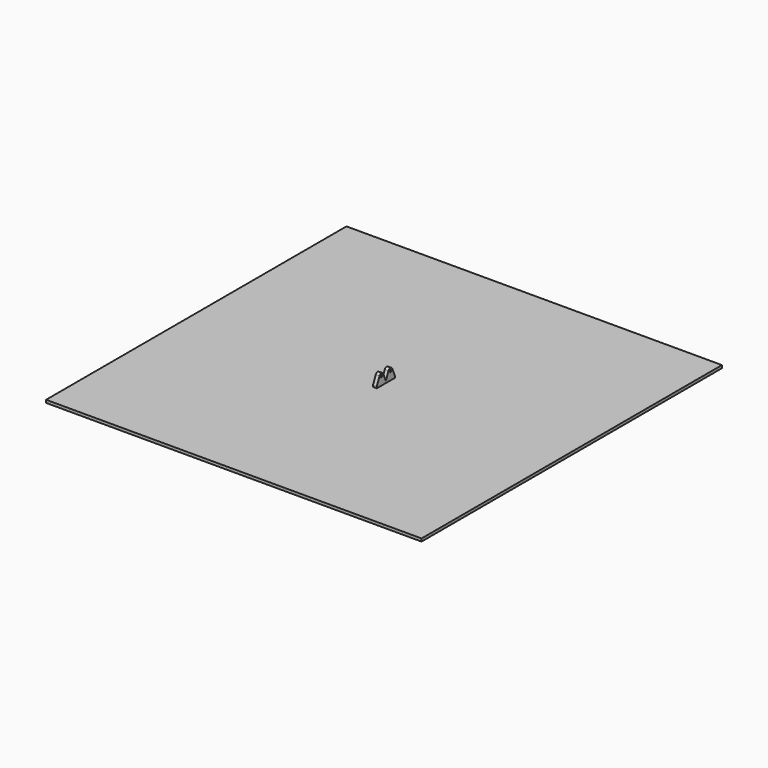
from build123d import *

# Parameters (mm, degrees)
F0_W     = 400
F0_H     = 400
F1_DEPTH = 3
F2_R     = 1.25
F2_W     = 12
F2_H     = 2
F3_DEPTH = 2
F4_DEPTH = 2


with BuildPart() as f1:
    # F0 (on Top) → F1 (new body)
    with BuildSketch(Plane.XY):
        Rectangle(F0_W, F0_H)
    extrude(amount=-F1_DEPTH)

    # F2 (on Right) → F3 (join)
    with BuildSketch(Plane.YZ):
        with BuildLine():
            ThreePointArc((-3.4732674635, 10.0854136027), (-6, 11.75), (-8.5267325365, 10.0854136027))
            ThreePointArc((-8.5267325365, 10.0854136027), (-6.5540692757, 6.3063951222), (-3.25, 9))
            ThreePointArc((-3.25, 9), (-3.3063951222, 9.5540692757), (-3.4732674635, 10.0854136027))
        make_face()
        with Locations((-6, 9)):
            Circle(F2_R, mode=Mode.SUBTRACT)
        with BuildLine():
            Line((-8.5267325365, 10.0854136027), (-12, 2))
            Line((-12, 2), (0, 2))
            Line((0, 2), (-3.4732674635, 10.0854136027))
            ThreePointArc((-3.4732674635, 10.0854136027), (-3.3063951222, 9.5540692757), (-3.25, 9))
            ThreePointArc((-3.25, 9), (-6.5540692757, 6.3063951222), (-8.5267325365, 10.0854136027))
        make_face()
        with Locations((-6, 1)):
            Rectangle(F2_W, F2_H)
        with Locations((6, 1)):
            Rectangle(F2_W, F2_H)
        with BuildLine():
            Line((3.4732674635, 10.0854136027), (0, 2))
            Line((0, 2), (12, 2))
            Line((12, 2), (8.5267325365, 10.0854136027))
            ThreePointArc((8.5267325365, 10.0854136027), (8.6936048778, 9.5540692757), (8.75, 9))
            ThreePointArc((8.75, 9), (5.4459307243, 6.3063951222), (3.4732674635, 10.0854136027))
        make_face()
        with BuildLine():
            ThreePointArc((8.5267325365, 10.0854136027), (6, 11.75), (3.4732674635, 10.0854136027))
            ThreePointArc((3.4732674635, 10.0854136027), (5.4459307243, 6.3063951222), (8.75, 9))
            ThreePointArc((8.75, 9), (8.6936048778, 9.5540692757), (8.5267325365, 10.0854136027))
        make_face()
        with Locations((6, 9)):
            Circle(F2_R, mode=Mode.SUBTRACT)
    extrude(amount=F3_DEPTH)

    # F4 (add): a face of the model
    f4_faces = [f1.faces().sort_by_distance(p)[0] for p in [
        (0, -6, 11.4827805209),
    ]]
    extrude(f4_faces, amount=F4_DEPTH)


solid = f1.part
